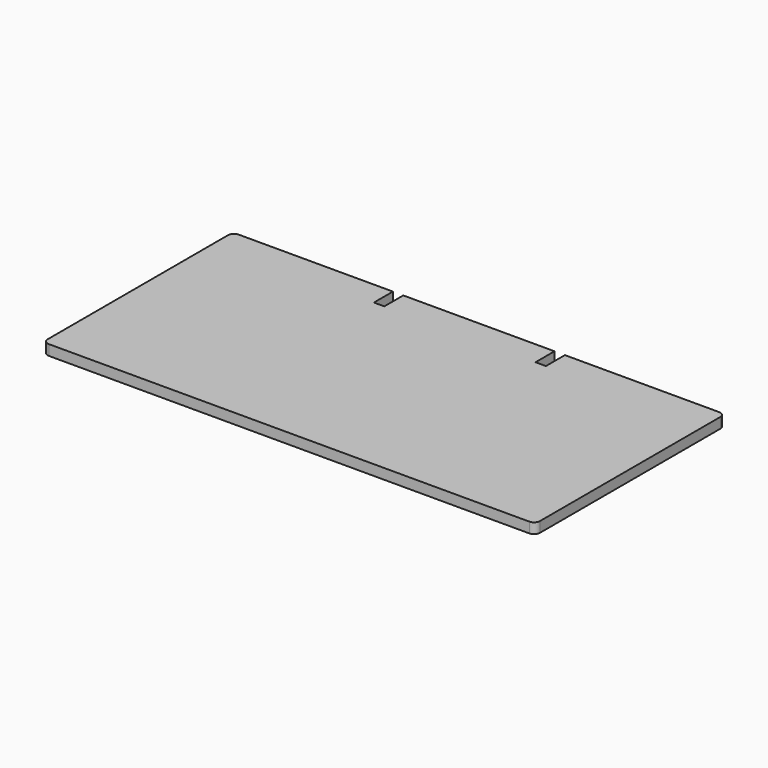
from build123d import *

# Parameters (mm, degrees)
F1_DEPTH = 11.1125
F2_R     = 6.35


# Not quite as in the source:
# - a feature names something its author has since deleted; it is built from what else it names


with BuildPart() as f1:
    # F0 (on Top) → F1 (new body)
    with BuildSketch(Plane.XY):
        Polygon((-263.525, -101.6), (-263.525, -127), (80.9498, -127), (92.075, -127), (263.525, -127), (263.525, -101.6), (263.525, 127), (92.075, 127), (92.075, 101.6), (80.9498, 101.6), (80.9498, 127), (-80.9498, 127), (-80.9498, 101.6), (-92.075, 101.6), (-92.075, 127), (-263.525, 127), align=None)
    extrude(amount=F1_DEPTH)

    # F2
    f2_edges = [f1.edges().sort_by_distance(p)[0] for p in [
        (263.525, -127, 5.55625),
        (263.525, 127, 5.55625),
        (-263.525, -127, 5.55625),
        (-263.525, 127, 5.55625),
    ]]
    fillet(f2_edges, radius=F2_R)


solid = f1.part
